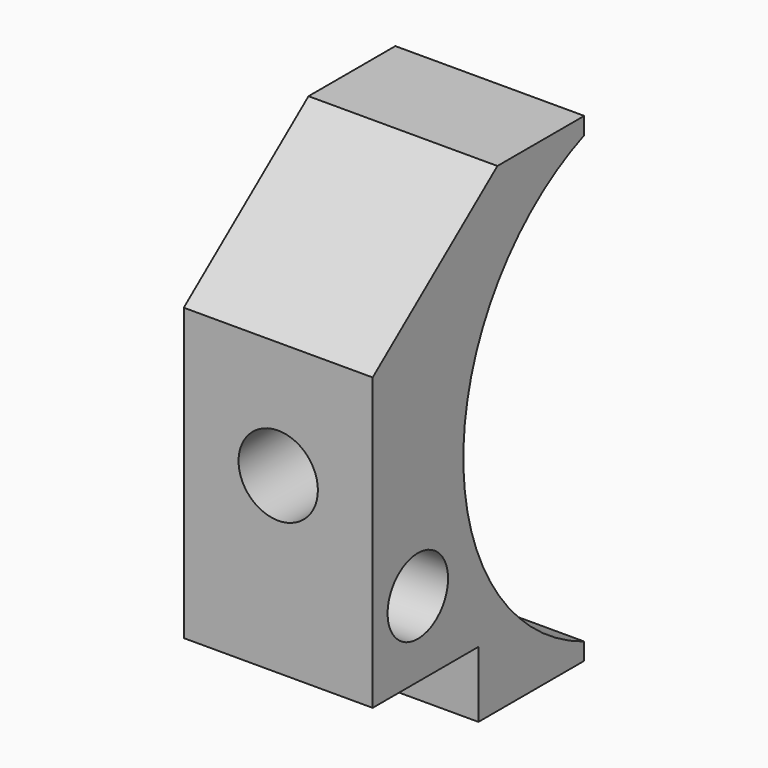
from build123d import *

# Parameters (mm, degrees)
F1_DEPTH = 14
F3_DEPTH = 11
F4_R     = 2.1
F5_DEPTH = 14.001
F6_SIZE2 = 6.5
F6_SIZE  = 8.255
F7_DEPTH = 25.4
F2_W     = 7
F2_H     = 3.5
F8_DEPTH = 10.0010001
F2_R     = 2
F9_DEPTH = 25


# Not quite as in the source:
# - a feature names something its author has since deleted; it is built from what else it names


with BuildPart() as f1:
    # F0 (on Front) → F1 (new body)
    with BuildSketch(Plane.XZ):
        Polygon((10, 21.0440813839), (0, 21.0440813839), (0, 0), (0, -4.3559186161), (10, -4.3559186161), (10, 0), align=None)
    extrude(amount=F1_DEPTH)

    # F2 (on face) → F3 (join)
    with BuildSketch(Plane.YZ.offset(10)):
        with BuildLine():
            Line((0, -3.4542235791), (0, 20.1423863469))
            ThreePointArc((0, 20.1423863469), (-8, 8.3440813839), (0, -3.4542235791))
        make_face()
    extrude(amount=-F3_DEPTH)

    # F4 (on face) → F5 (cut, through all)
    with BuildSketch(Plane.XZ.offset(14)):
        with Locations((5, 8.3440813839)):
            Circle(F4_R)
    extrude(amount=-F5_DEPTH, mode=Mode.SUBTRACT)

    # F6
    f6_edges = [f1.edges().sort_by_distance(p)[0] for p in [
        (5, -14, 21.044081),
    ]]
    f6_side = f1.faces().sort_by_distance((5, -7, 21.044081))[0]
    chamfer(f6_edges, length=F6_SIZE, length2=F6_SIZE2, reference=f6_side)

    # F2 (on face) → F7 (cut)
    with BuildSketch(Plane.YZ.offset(10)):
        with BuildLine():
            Line((0, -3.4542235791), (0, 20.1423863469))
            ThreePointArc((0, 20.1423863469), (-8, 8.3440813839), (0, -3.4542235791))
        make_face()
    extrude(amount=-F7_DEPTH, mode=Mode.SUBTRACT)

    # F2 (on face) → F8 (cut, through all)
    with BuildSketch(Plane.YZ.offset(10)):
        with Locations((-10.5, -2.6059186161)):
            Rectangle(F2_W, F2_H)
    extrude(amount=-F8_DEPTH, mode=Mode.SUBTRACT)

    # F2 (on face) → F9 (cut)
    with BuildSketch(Plane.YZ.offset(10)):
        with BuildLine():
            Line((4.7, 21.0440813839), (1.525, 21.0440813839))
            Line((1.525, 21.0440813839), (1.525, 20.6408035082))
            ThreePointArc((1.525, 20.6408035082), (3.0997454855, 20.9428585265), (4.7, 21.0440813839))
        make_face()
        with BuildLine():
            Line((7.875, 21.0440813839), (4.7, 21.0440813839))
            ThreePointArc((4.7, 21.0440813839), (3.0997454855, 20.9428585265), (1.525, 20.6408035082))
            Line((1.525, 20.6408035082), (1.525, -3.9526407403))
            ThreePointArc((1.525, -3.9526407403), (3.0997454855, -4.2546957586), (4.7, -4.3559186161))
            Line((4.7, -4.3559186161), (7.875, -4.3559186161))
            Line((7.875, -4.3559186161), (7.875, 21.0440813839))
        make_face()
        with BuildLine():
            Line((1.525, -3.9526407403), (1.525, 20.6408035082))
            ThreePointArc((1.525, 20.6408035082), (0.7546215433, 20.4157005311), (0, 20.1423863469))
            Line((0, 20.1423863469), (0, -3.4542235791))
            ThreePointArc((0, -3.4542235791), (0.7546215433, -3.7275377632), (1.525, -3.9526407403))
        make_face()
        with BuildLine():
            ThreePointArc((4.7, -4.3559186161), (3.0997454855, -4.2546957586), (1.525, -3.9526407403))
            Line((1.525, -3.9526407403), (1.525, -4.3559186161))
            Line((1.525, -4.3559186161), (2.607938957, -4.3559186161))
            Line((2.607938957, -4.3559186161), (4.7, -4.3559186161))
        make_face()
        with BuildLine():
            Line((0, -3.4542235791), (0, 20.1423863469))
            ThreePointArc((0, 20.1423863469), (-8, 8.3440813839), (0, -3.4542235791))
        make_face()
        with Locations((-11.0123908797, 3.1440813839)):
            Circle(F2_R)
    extrude(amount=-F9_DEPTH, mode=Mode.SUBTRACT)


solid = f1.part
